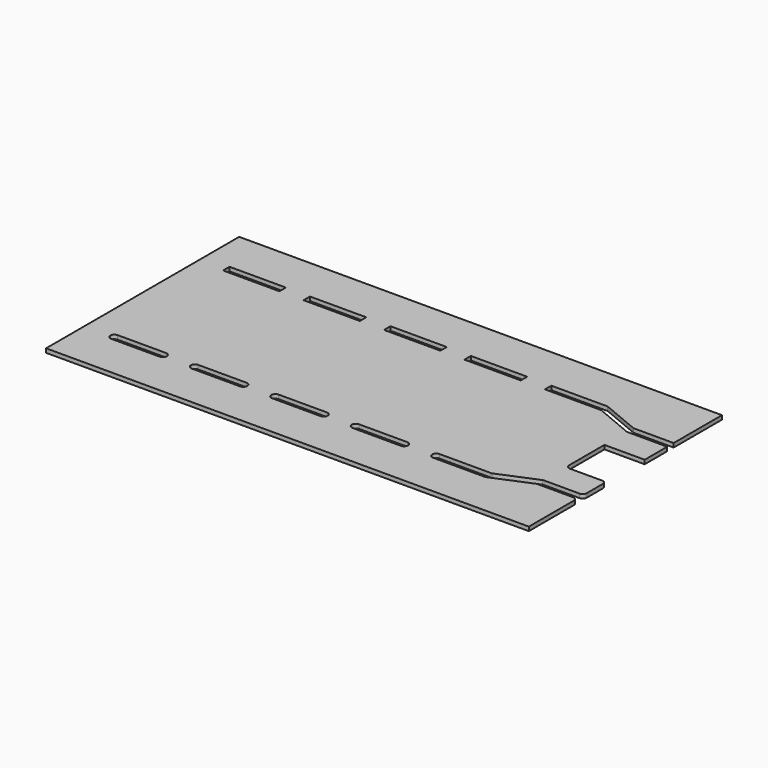
from build123d import *

# Parameters (mm, degrees)
F0_W     = 70
F0_H     = 10
F1_DEPTH = 5
F2_R     = 4.99999


# Not quite as in the source:
# - a fillet or chamfer is up to 0.001 mm smaller than in the source, because OpenCascade refuses the exact size


with BuildPart() as f1:
    # F0 (on Top) → F1 (new body)
    with BuildSketch(Plane.XY):
        Polygon((300, 149.2274475843), (-300, 149.2274475843), (-300, -150.7725524157), (300, -150.7725524157), (300, -75.7725524157), (250, -75.7725524157), (201.9998562336, -95.7725524157), (131.9998562336, -95.7725524157), (131.9998562336, -85.7725524157), (201.9998562336, -85.7725524157), (250, -65.7725524157), (300, -65.7725524157), (300, -30.7725524157), (250, -30.7725524157), (250, 29.2274475843), (300, 29.2274475843), (300, 64.2274475843), (250, 64.2274475843), (201.9998562336, 84.2274475843), (131.9998562336, 84.2274475843), (131.9998562336, 94.2274475843), (201.9998562336, 94.2274475843), (250, 74.2274475843), (300, 74.2274475843), align=None)
        with Locations((-233.0001437664, -90.7725524157)):
            Rectangle(F0_W, F0_H, mode=Mode.SUBTRACT)
        with Locations((-133.0001437664, -90.7725524157)):
            Rectangle(F0_W, F0_H, mode=Mode.SUBTRACT)
        with Locations((-33.0001437664, -90.7725524157)):
            Rectangle(F0_W, F0_H, mode=Mode.SUBTRACT)
        with Locations((66.9998562336, -90.7725524157)):
            Rectangle(F0_W, F0_H, mode=Mode.SUBTRACT)
        with Locations((-233.0001437664, 89.2274475843)):
            Rectangle(F0_W, F0_H, mode=Mode.SUBTRACT)
        with Locations((-133.0001437664, 89.2274475843)):
            Rectangle(F0_W, F0_H, mode=Mode.SUBTRACT)
        with Locations((-33.0001437664, 89.2274475843)):
            Rectangle(F0_W, F0_H, mode=Mode.SUBTRACT)
        with Locations((66.9998562336, 89.2274475843)):
            Rectangle(F0_W, F0_H, mode=Mode.SUBTRACT)
    extrude(amount=F1_DEPTH)

    # F2 (radius 5 in the source; OpenCascade refuses exactly that, so slightly less here)
    f2_edges = [f1.edges().sort_by_distance(p)[0] for p in [
        (131.999856, -95.772552, 2.5),
        (31.999856, -95.772552, 2.5),
        (-68.000144, -95.772552, 2.5),
        (201.999856, -95.772552, 2.5),
        (250, -75.772552, 2.5),
        (-168.000144, -95.772552, 2.5),
        (-268.000144, -95.772552, 2.5),
        (300, -75.772552, 2.5),
        (300, -65.772552, 2.5),
        (300, -30.772552, 2.5),
        (250, -30.772552, 2.5),
        (250, -65.772552, 2.5),
        (201.999856, -85.772552, 2.5),
        (131.999856, -85.772552, 2.5),
        (101.999856, -85.772552, 2.5),
        (1.999856, -85.772552, 2.5),
        (-98.000144, -85.772552, 2.5),
        (-198.000144, -85.772552, 2.5),
        (31.999856, -85.772552, 2.5),
        (-68.000144, -85.772552, 2.5),
        (-168.000144, -85.772552, 2.5),
        (-268.000144, -85.772552, 2.5),
        (101.999856, -95.772552, 2.5),
        (1.999856, -95.772552, 2.5),
        (-98.000144, -95.772552, 2.5),
        (-198.000144, -95.772552, 2.5),
    ]]
    fillet(f2_edges, radius=F2_R)


solid = f1.part
